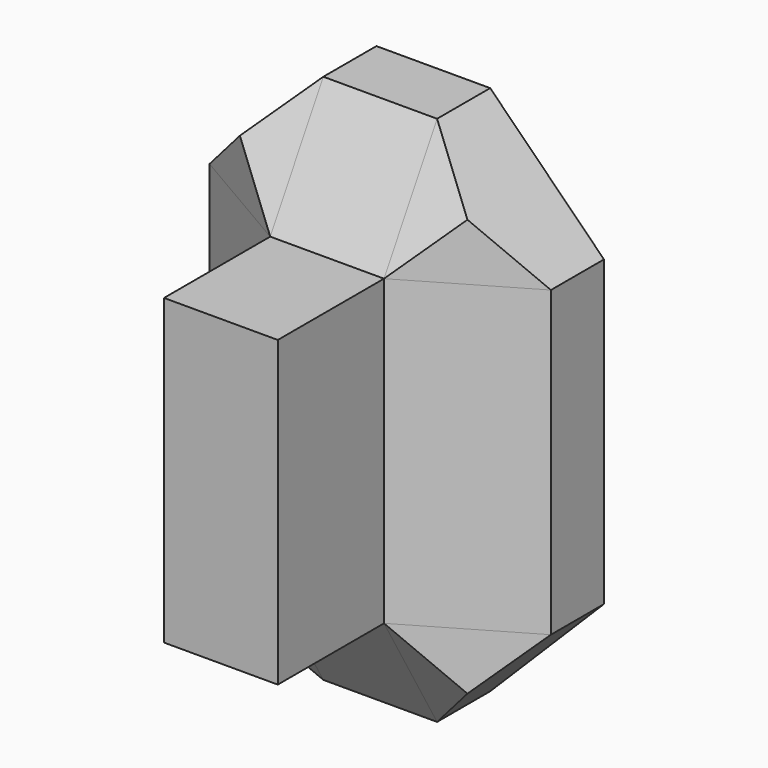
from build123d import *

# Parameters (mm, degrees)
F0_W          = 15
F0_H          = 8.75
F0_H_2        = 17.5
F1_DEPTH      = 40
F2_DEPTH      = 55
F3_DEPTH      = 15
F7_DEPTH      = 20.4590409994
F8_ANGLE      = 180
F10_DEPTH     = 25
F11_T4_DEPTH  = 56.0752448195
F11_T12_DEPTH = 56.0752448195
F11_T20_DEPTH = 56.0752448195
F11_T28_DEPTH = 56.0752448195


# Not quite as in the source:
# - a fillet or chamfer that OpenCascade refuses, or shapes differently, is made with other operations: its cross-section is extruded or revolved along the edge and cut away or added


with BuildPart() as f1:
    # F0 (on Top) → F1 (new body)
    with BuildSketch(Plane.XY):
        with Locations((0, 13.125)):
            Rectangle(F0_W, F0_H)
        with Locations((0, -8.75)):
            Rectangle(F0_W, F0_H_2)
        with Locations((0, 4.375)):
            Rectangle(F0_W, F0_H)
        with Locations((15, 13.125)):
            Rectangle(F0_W, F0_H)
        Polygon((22.5, 8.75), (7.5, 8.75), (7.5, 0), align=None)
        with Locations((-15, 13.125)):
            Rectangle(F0_W, F0_H)
        Polygon((-7.5, 0), (-7.5, 8.75), (-22.5, 8.75), align=None)
    extrude(amount=F1_DEPTH)



with BuildPart() as f2:
    # F0 (on Top) → F2 (new body)
    with BuildSketch(Plane.XY):
        with Locations((0, 4.375)):
            Rectangle(F0_W, F0_H)
        with Locations((0, 13.125)):
            Rectangle(F0_W, F0_H)
    extrude(amount=F2_DEPTH)


with BuildPart() as f1_1:
    add(f1.part)

    add(f2.part)  # F3 merges F2
    # F0 (on Top) → F3 (join)
    with BuildSketch(Plane.XY):
        with Locations((0, 4.375)):
            Rectangle(F0_W, F0_H)
        with Locations((0, 13.125)):
            Rectangle(F0_W, F0_H)
    extrude(amount=-F3_DEPTH)

    # F4: union 


with BuildPart() as f1_2:
    # F6: moved
    add(f1_1.part.moved(Location((7.5, 0, 0))))

    # F5 (on Right) → F7 (cut)
    with BuildSketch(Plane.YZ):
        Polygon((8.75, -15), (0, 0), (0, -15), align=None)
    extrude(amount=F7_DEPTH, mode=Mode.SUBTRACT)


with BuildPart() as f1_3:
    # F8: moved
    add(f1_2.part.rotate(Axis((7.5, 0, 0), (0, -1, 0)), F8_ANGLE))


with BuildPart() as f1_4:
    # F9: moved
    add(f1_3.part.moved(Location((0, 0, 40))))

    # F5 (on Right) → F10 (cut)
    with BuildSketch(Plane.YZ):
        Polygon((8.75, -15), (0, 0), (0, -15), align=None)
    extrude(amount=F10_DEPTH, mode=Mode.SUBTRACT)

    # F11: chamfer of 15 on 4 edges, made by hand


with BuildPart() as f11_tool2:
    # F11_s3 → F11_t4 (new body)
    with BuildSketch(Plane.XZ.offset(-17.5)):
        Polygon((30, 40), (15, 55), (15, 40), align=None)
    extrude(amount=F11_T4_DEPTH)

    split(bisect_by=Plane.YZ.offset(30), keep=Keep.BOTTOM)

    split(bisect_by=Plane(origin=(3.8082901554, -6.5284974093, 0), x_dir=(0, 0, 1), z_dir=(-0.5038710255, 0.8637789009, 0)), keep=Keep.TOP)

    split(bisect_by=Plane(origin=(0, -17.4093264249, 10.1554404145), x_dir=(1, 0, 0), z_dir=(0, 0.8637789009, -0.5038710255)), keep=Keep.TOP)

    split(bisect_by=Plane.XY.offset(55), keep=Keep.BOTTOM)


with BuildPart() as f1_5:
    add(f1_4.part)

    # F11_t1: union F11_tool2
    add(f11_tool2.part)


with BuildPart() as f11_tool10:
    # F11_s11 → F11_t12 (new body)
    with BuildSketch(Plane.XZ.offset(38.5752448195)):
        Polygon((-15, 0), (0, -15), (0, 0), align=None)
    extrude(amount=-F11_T12_DEPTH)

    split(bisect_by=Plane.YZ.offset(-15), keep=Keep.TOP)

    split(bisect_by=Plane(origin=(0, 0, 0), x_dir=(0, 0, 1), z_dir=(0.5038710255, 0.8637789009, 0)), keep=Keep.TOP)

    split(bisect_by=Plane.XY.offset(-15), keep=Keep.TOP)

    split(bisect_by=Plane(origin=(0, 0, 0), x_dir=(1, 0, 0), z_dir=(0, 0.8637789009, 0.5038710255)), keep=Keep.TOP)


with BuildPart() as f1_6:
    add(f1_5.part)

    # F11_t9: union F11_tool10
    add(f11_tool10.part)


with BuildPart() as f11_tool18:
    # F11_s19 → F11_t20 (new body)
    with BuildSketch(Plane.XZ.offset(-17.5)):
        Polygon((15, -15), (30, 0), (15, 0), align=None)
    extrude(amount=F11_T20_DEPTH)

    split(bisect_by=Plane.XY.offset(-15), keep=Keep.TOP)

    split(bisect_by=Plane(origin=(0, 0, 0), x_dir=(1, 0, 0), z_dir=(0, 0.8637789009, 0.5038710255)), keep=Keep.TOP)

    split(bisect_by=Plane(origin=(3.8082901554, -6.5284974093, 0), x_dir=(0, 0, 1), z_dir=(-0.5038710255, 0.8637789009, 0)), keep=Keep.TOP)

    split(bisect_by=Plane.YZ.offset(30), keep=Keep.BOTTOM)


with BuildPart() as f1_7:
    add(f1_6.part)

    # F11_t17: union F11_tool18
    add(f11_tool18.part)


with BuildPart() as f11_tool26:
    # F11_s27 → F11_t28 (new body)
    with BuildSketch(Plane.XZ.offset(38.5752448195)):
        Polygon((0, 55), (-15, 40), (0, 40), align=None)
    extrude(amount=-F11_T28_DEPTH)

    split(bisect_by=Plane.XY.offset(55), keep=Keep.BOTTOM)

    split(bisect_by=Plane(origin=(0, -17.4093264249, 10.1554404145), x_dir=(1, 0, 0), z_dir=(0, 0.8637789009, -0.5038710255)), keep=Keep.TOP)

    split(bisect_by=Plane.YZ.offset(-15), keep=Keep.TOP)

    split(bisect_by=Plane(origin=(0, 0, 0), x_dir=(0, 0, 1), z_dir=(0.5038710255, 0.8637789009, 0)), keep=Keep.TOP)


with BuildPart() as f1_8:
    add(f1_7.part)

    # F11_t25: union F11_tool26
    add(f11_tool26.part)


solid = f1_8.part
